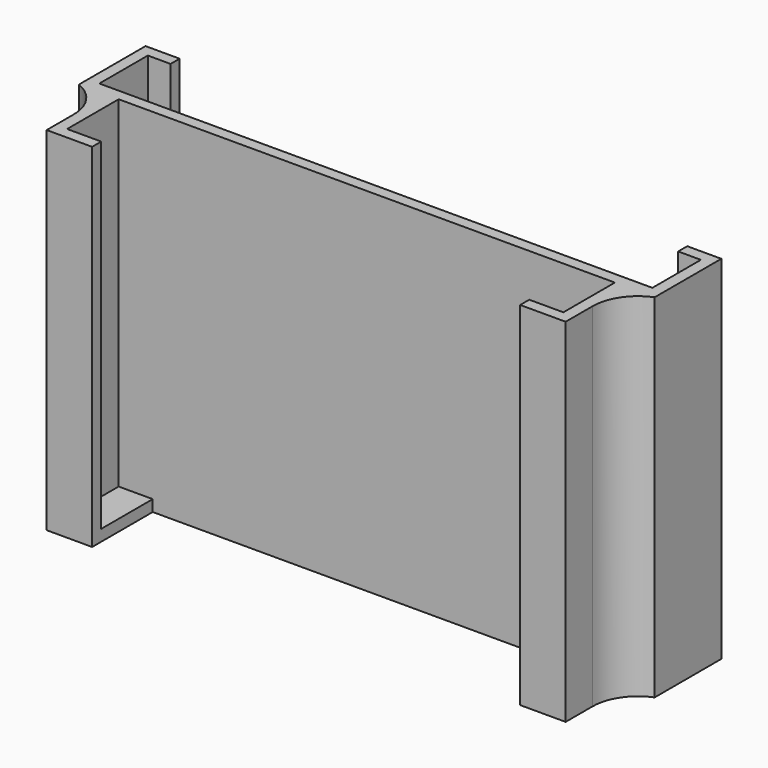
from build123d import *

# Parameters (mm, degrees)
F1_DEPTH    = 45
F2_T1_DEPTH = 45
F3_W        = 4.5
F3_H        = 8.5
F4_DEPTH    = 1.5


# Not quite as in the source:
# - a fillet or chamfer that OpenCascade refuses, or shapes differently, is made with other operations: its cross-section is extruded or revolved along the edge and cut away or added


with BuildPart() as f1:
    # F0 (on Top) → F1 (new body)
    with BuildSketch(Plane.XY):
        Polygon((36.5, 0), (0, 0), (-36.5, 0), (-36.5, 8), (-33.5, 8), (-33.5, 9.5), (-38, 9.5), (-38, -1.5), (-34.25, -1.5), (-32.75, -1.5), (0, -1.5), (32.75, -1.5), (34.25, -1.5), (38, -1.5), (38, 9.5), (33.5, 9.5), (33.5, 8), (36.5, 8), align=None)
        Polygon((-32.75, -1.5), (-34.25, -1.5), (-34.25, -11.5), (-28.25, -11.5), (-28.25, -10), (-32.75, -10), align=None)
        Polygon((34.25, -11.5), (34.25, -1.5), (32.75, -1.5), (32.75, -10), (28.25, -10), (28.25, -11.5), align=None)
    extrude(amount=F1_DEPTH)

    # F2: fillet of radius 6 on 2 edges, made by hand

    # F2_s2 → F2_t1 (join)
    with BuildSketch(Plane.XY):
        with BuildLine():
            ThreePointArc((-38, -1.5), (-35.2750628145, -3.7080468991), (-34.25, -7.0621488653))
            Line((-34.25, -7.0621488653), (-34.25, -1.5))
            Line((-34.25, -1.5), (-38, -1.5))
        make_face()
        with BuildLine():
            ThreePointArc((34.25, -7.0621488653), (35.2750628145, -3.7080468991), (38, -1.5))
            Line((38, -1.5), (34.25, -1.5))
            Line((34.25, -1.5), (34.25, -7.0621488653))
        make_face()
    extrude(amount=F2_T1_DEPTH)

    # F3 (on face) → F4 (join)
    with BuildSketch(Plane(origin=(0, 0, 0), x_dir=(1, 0, 0), z_dir=(0, 0, -1))):
        with BuildLine():
            Line((-32.75, 10), (-28.25, 10))
            Line((-28.25, 10), (-28.25, 11.5))
            Line((-28.25, 11.5), (-34.25, 11.5))
            Line((-34.25, 11.5), (-34.25, 7.0621488653))
            ThreePointArc((-34.25, 7.0621488653), (-35.2750628145, 3.7080468991), (-38, 1.5))
            Line((-38, 1.5), (-38, -9.5))
            Line((-38, -9.5), (-33.5, -9.5))
            Line((-33.5, -9.5), (-33.5, -8))
            Line((-33.5, -8), (-36.5, -8))
            Line((-36.5, -8), (-36.5, 0))
            Line((-36.5, 0), (-28, 0))
            Line((-28, 0), (20, 0))
            Line((20, 0), (36.5, 0))
            Line((36.5, 0), (36.5, -8))
            Line((36.5, -8), (33.5, -8))
            Line((33.5, -8), (33.5, -9.5))
            Line((33.5, -9.5), (38, -9.5))
            Line((38, -9.5), (38, 1.5))
            ThreePointArc((38, 1.5), (35.2750628145, 3.7080468991), (34.25, 7.0621488653))
            Line((34.25, 7.0621488653), (34.25, 11.5))
            Line((34.25, 11.5), (28.25, 11.5))
            Line((28.25, 11.5), (28.25, 10))
            Line((28.25, 10), (32.75, 10))
            Line((32.75, 10), (32.75, 1.5))
            Line((32.75, 1.5), (28.25, 1.5))
            Line((28.25, 1.5), (-28.25, 1.5))
            Line((-28.25, 1.5), (-32.75, 1.5))
            Line((-32.75, 1.5), (-32.75, 10))
        make_face()
        with Locations((-30.5, 5.75)):
            Rectangle(F3_W, F3_H)
        Polygon((-33.5, -8), (-33.5, -9.5), (-28, -9.5), (-28, 0), (-36.5, 0), (-36.5, -8), align=None)
        with Locations((30.5, 5.75)):
            Rectangle(F3_W, F3_H)
        Polygon((20, -9.5), (33.5, -9.5), (33.5, -8), (36.5, -8), (36.5, 0), (20, 0), align=None)
    extrude(amount=F4_DEPTH)


solid = f1.part
